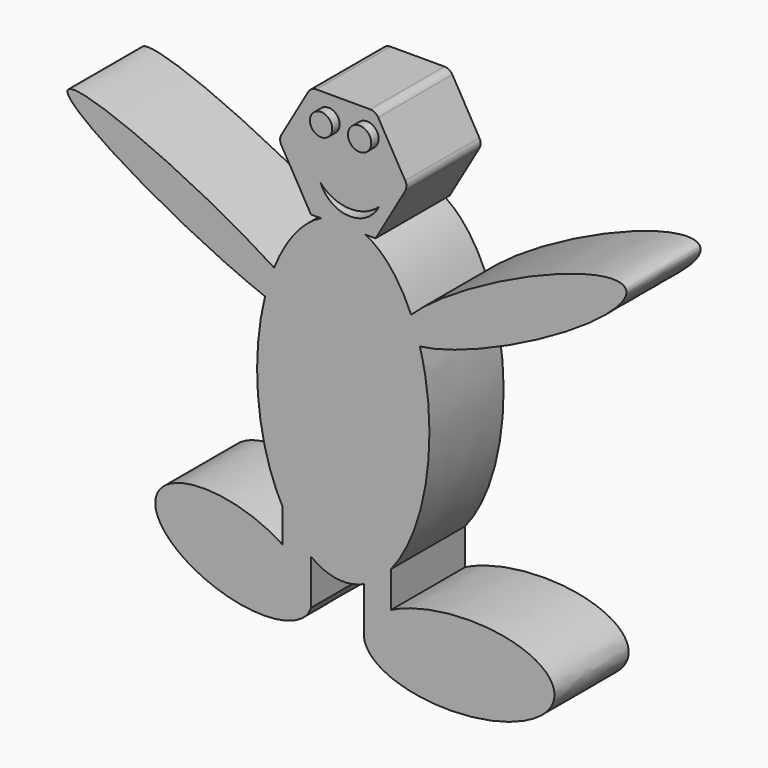
from build123d import *

# Parameters (mm, degrees)
F1_DEPTH = 50
F2_R     = 6.0155907658
F2_R_2   = 6.2756136539
F3_DEPTH = 5
F4_DEPTH = 10
F5_R     = 5
F7_DEPTH = 50


with BuildPart() as f1:
    # F0 (on Front) → F1 (new body)
    with BuildSketch(Plane.XZ):
        Polygon((17.4143397291, 30.1625211911), (-17.4143397291, 30.1625211911), (-34.8286794583, 0), (-17.4143397291, -30.1625211911), (17.4143397291, -30.1625211911), (34.8286794583, 0), align=None)
    extrude(amount=F1_DEPTH)

    # F2 (on face) → F3 (join)
    with BuildSketch(Plane.XZ.offset(50)):
        with Locations((-7.967392914, 17.6304206252)):
            Circle(F2_R)
        with Locations((12.811797671, 17.6304578781)):
            Circle(F2_R_2)
    extrude(amount=F3_DEPTH)

    # F2 (on face) → F4 (cut)
    with BuildSketch(Plane.XZ.offset(50)):
        with BuildLine():
            ThreePointArc((19.3255450577, -14.4387213513), (3.3384184901, -20.5933298221), (-12.2403670102, -13.468102552))
            ThreePointArc((-12.2403670102, -13.468102552), (3.2273641474, -24.2049759369), (19.3255450577, -14.4387213513))
        make_face()
    extrude(amount=-F4_DEPTH, mode=Mode.SUBTRACT)

    # F5
    f5_edges = [f1.edges().sort_by_distance(p)[0] for p in [
        (17.41434, -25, 30.162521),
        (-17.41434, -25, 30.162521),
        (34.828679, -25, 0),
        (-34.828679, -25, 0),
    ]]
    fillet(f5_edges, radius=F5_R)

    # F6 (on Front) → F7 (join)
    with BuildSketch(Plane.XZ):
        with BuildLine():
            add(Edge.make_bspline(
                [(41.2922416881, -73.6853662735), (169.4693590378, -59.4246752204), (152.5160927466, -10.667922077), (135.5628264553, 38.0888310665), (36.5988004625, -60.1872620557)],
                knots=[0.5054493336, 0.5054493336, 0.5054493336, 3.1146139618, 3.1146139618, 5.7237785899, 5.7237785899, 5.7237785899], degree=2, weights=[1, 0.2630807094, 1, 0.2630807094, 1]))
            add(Edge.make_bspline(
                [(41.2922416881, -73.6853662735), (39.2889405165, -66.529639937), (36.5988004625, -60.1872620557)],
                knots=[5.1892655065, 5.1892655065, 5.1892655065, 5.376524204, 5.376524204, 5.376524204], degree=2, weights=[1, 0.9956199737, 1]))
        make_face()
        with BuildLine():
            add(Edge.make_bspline(
                [(-37.2982655111, -61.8791791625), (-40.1784962307, -69.0282916237), (-42.20112137, -77.1171546989)],
                knots=[0.9314728887, 0.9314728887, 0.9314728887, 1.1384572321, 1.1384572321, 1.1384572321], degree=2, weights=[1, 0.9946494634, 1]))
            add(Edge.make_bspline(
                [(-37.2982655111, -61.8791791625), (-142.2676835981, 6.0363373075), (-148.6893936246, -13.9222058565), (-155.1111036512, -33.8807490205), (-42.20112137, -77.1171546989)],
                knots=[0.9261808498, 0.9261808498, 0.9261808498, 3.1635032717, 3.1635032717, 5.4008256936, 5.4008256936, 5.4008256936], degree=2, weights=[1, 0.4368871001, 1, 0.4368871001, 1]))
        make_face()
        with BuildLine():
            add(Edge.make_bspline(
                [(36.5988004625, -60.1872620557), (22.6424707083, -27.2832810879), (0, -27.2832810879)],
                knots=[5.376524204, 5.376524204, 5.376524204, 6.2831853072, 6.2831853072, 6.2831853072], degree=2, weights=[1, 0.8989934357, 1]))
            add(Edge.make_bspline(
                [(0, -27.2832810879), (-23.3602880424, -27.2832810879), (-37.2982655111, -61.8791791625)],
                knots=[0, 0, 0, 0.9314728887, 0.9314728887, 0.9314728887], degree=2, weights=[1, 0.8934910848, 1]))
            add(Edge.make_bspline(
                [(-14.1357605669, -82.8124405083), (-11.8424071187, -78.3491930143), (-37.2982655111, -61.8791791625)],
                knots=[0, 0, 0, 0.9261808498, 0.9261808498, 0.9261808498], degree=2, weights=[1, 0.8946762325, 1]))
            add(Edge.make_bspline(
                [(-42.20112137, -77.1171546989), (-16.3047277649, -87.0336116578), (-14.1357605669, -82.8124405083)],
                knots=[5.4008256936, 5.4008256936, 5.4008256936, 6.2831853072, 6.2831853072, 6.2831853072], degree=2, weights=[1, 0.9042485074, 1]))
            add(Edge.make_bspline(
                [(-42.20112137, -77.1171546989), (-55.8693379467, -131.7789554553), (-32.6593779027, -174.0816324883)],
                knots=[1.1384572321, 1.1384572321, 1.1384572321, 2.3624206627, 2.3624206627, 2.3624206627], degree=2, weights=[1, 0.8185111489, 1]))
            Line((-32.6593779027, -174.0816324883), (-32.6593779027, -169.5833057165))
            Line((-32.6593779027, -169.5833057165), (-17.4256470054, -169.5833057165))
            Line((-17.4256470054, -169.5833057165), (-17.4256470054, -192.5705769551))
            add(Edge.make_bspline(
                [(-17.4256470054, -192.5705769551), (-3.4362621433, -203.0115231159), (11.2084979191, -196.2957137528)],
                knots=[2.7572761224, 2.7572761224, 2.7572761224, 3.3851526537, 3.3851526537, 3.3851526537], degree=2, weights=[1, 0.9511247857, 1]))
            Line((11.2084979191, -196.2957137528), (11.2084979191, -181.6708147526))
            Line((11.2084979191, -181.6708147526), (25.7280766964, -181.6708147526))
            Line((25.7280766964, -181.6708147526), (25.7280766964, -184.4870319799))
            add(Edge.make_bspline(
                [(25.7280766964, -184.4870319799), (60.4040061865, -141.9519646735), (41.2922416881, -73.6853662735)],
                knots=[3.7282237262, 3.7282237262, 3.7282237262, 5.1892655065, 5.1892655065, 5.1892655065], degree=2, weights=[1, 0.7448269354, 1]))
            add(Edge.make_bspline(
                [(30.647560719, -71.4679593328), (32.2659775962, -74.6896076408), (41.2922416881, -73.6853662735)],
                knots=[0, 0, 0, 0.5054493336, 0.5054493336, 0.5054493336], degree=2, weights=[1, 0.9682347327, 1]))
            add(Edge.make_bspline(
                [(36.5988004625, -60.1872620557), (28.8474842086, -67.884696253), (30.647560719, -71.4679593328)],
                knots=[5.7237785899, 5.7237785899, 5.7237785899, 6.2831853072, 6.2831853072, 6.2831853072], degree=2, weights=[1, 0.9611373745, 1]))
        make_face()
        with BuildLine():
            add(Edge.make_bspline(
                [(41.2922416881, -73.6853662735), (39.2889405165, -66.529639937), (36.5988004625, -60.1872620557)],
                knots=[5.1892655065, 5.1892655065, 5.1892655065, 5.376524204, 5.376524204, 5.376524204], degree=2, weights=[1, 0.9956199737, 1]))
            add(Edge.make_bspline(
                [(36.5988004625, -60.1872620557), (28.8474842086, -67.884696253), (30.647560719, -71.4679593328)],
                knots=[5.7237785899, 5.7237785899, 5.7237785899, 6.2831853072, 6.2831853072, 6.2831853072], degree=2, weights=[1, 0.9611373745, 1]))
            add(Edge.make_bspline(
                [(30.647560719, -71.4679593328), (32.2659775962, -74.6896076408), (41.2922416881, -73.6853662735)],
                knots=[0, 0, 0, 0.5054493336, 0.5054493336, 0.5054493336], degree=2, weights=[1, 0.9682347327, 1]))
        make_face()
        with BuildLine():
            add(Edge.make_bspline(
                [(-14.1357605669, -82.8124405083), (-11.8424071187, -78.3491930143), (-37.2982655111, -61.8791791625)],
                knots=[0, 0, 0, 0.9261808498, 0.9261808498, 0.9261808498], degree=2, weights=[1, 0.8946762325, 1]))
            add(Edge.make_bspline(
                [(-37.2982655111, -61.8791791625), (-40.1784962307, -69.0282916237), (-42.20112137, -77.1171546989)],
                knots=[0.9314728887, 0.9314728887, 0.9314728887, 1.1384572321, 1.1384572321, 1.1384572321], degree=2, weights=[1, 0.9946494634, 1]))
            add(Edge.make_bspline(
                [(-42.20112137, -77.1171546989), (-16.3047277649, -87.0336116578), (-14.1357605669, -82.8124405083)],
                knots=[5.4008256936, 5.4008256936, 5.4008256936, 6.2831853072, 6.2831853072, 6.2831853072], degree=2, weights=[1, 0.9042485074, 1]))
        make_face()
        with BuildLine():
            Line((-32.6593779027, -169.5833057165), (-32.6593779027, -174.0816324883))
            add(Edge.make_bspline(
                [(-32.6593779027, -174.0816324883), (-26.0445481198, -186.1378793499), (-17.4256470054, -192.5705769551)],
                knots=[2.3624206627, 2.3624206627, 2.3624206627, 2.7572761224, 2.7572761224, 2.7572761224], degree=2, weights=[1, 0.9805743661, 1]))
            Line((-17.4256470054, -192.5705769551), (-17.4256470054, -169.5833057165))
            Line((-17.4256470054, -169.5833057165), (-32.6593779027, -169.5833057165))
        make_face()
        with BuildLine():
            add(Edge.make_bspline(
                [(-32.6593779027, -174.0816324883), (-26.0445481198, -186.1378793499), (-17.4256470054, -192.5705769551)],
                knots=[2.3624206627, 2.3624206627, 2.3624206627, 2.7572761224, 2.7572761224, 2.7572761224], degree=2, weights=[1, 0.9805743661, 1]))
            Line((-32.6593779027, -174.0816324883), (-32.6593779027, -191.9202000812))
            add(Edge.make_bspline(
                [(-17.4256470054, -209.6746091398), (-19.9783918544, -200.3396941884), (-32.6593779027, -191.9202000812)],
                knots=[0.3149352399, 0.3149352399, 0.3149352399, 1.0505459948, 1.0505459948, 1.0505459948], degree=2, weights=[1, 0.9331187091, 1]))
            Line((-17.4256470054, -209.6746091398), (-17.4256470054, -192.5705769551))
        make_face()
        with BuildLine():
            add(Edge.make_bspline(
                [(-17.4256470054, -209.6746091398), (-19.9783918544, -200.3396941884), (-32.6593779027, -191.9202000812)],
                knots=[0.3149352399, 0.3149352399, 0.3149352399, 1.0505459948, 1.0505459948, 1.0505459948], degree=2, weights=[1, 0.9331187091, 1]))
            Line((-32.6593779027, -191.9202000812), (-32.6593779027, -216.8934494257))
            Line((-32.6593779027, -216.8934494257), (-17.4256470054, -216.8934494257))
            Line((-17.4256470054, -216.8934494257), (-17.4256470054, -209.6746091398))
        make_face()
        with BuildLine():
            Line((-32.6593779027, -216.8934494257), (-32.6593779027, -191.9202000812))
            add(Edge.make_bspline(
                [(-32.6593779027, -191.9202000812), (-155.0656797466, -110.6489855928), (-98.566158617, -203.2708546887), (-42.0666374873, -295.8927237846), (-17.4256470054, -216.8934494257)],
                knots=[1.0505459948, 1.0505459948, 1.0505459948, 3.666865651, 3.666865651, 6.2831853072, 6.2831853072, 6.2831853072], degree=2, weights=[1, 0.2596275414, 1, 0.2596275414, 1]))
            Line((-17.4256470054, -216.8934494257), (-32.6593779027, -216.8934494257))
        make_face()
        with BuildLine():
            add(Edge.make_bspline(
                [(11.2084979191, -196.2957137528), (19.0225466962, -192.7123391043), (25.7280766964, -184.4870319799)],
                knots=[3.3851526537, 3.3851526537, 3.3851526537, 3.7282237262, 3.7282237262, 3.7282237262], degree=2, weights=[1, 0.9853238194, 1]))
            Line((25.7280766964, -184.4870319799), (25.7280766964, -181.6708147526))
            Line((25.7280766964, -181.6708147526), (11.2084979191, -181.6708147526))
            Line((11.2084979191, -181.6708147526), (11.2084979191, -196.2957137528))
        make_face()
        with BuildLine():
            Line((25.7280766964, -203.876795604), (25.7280766964, -184.4870319799))
            add(Edge.make_bspline(
                [(11.2084979191, -196.2957137528), (19.0225466962, -192.7123391043), (25.7280766964, -184.4870319799)],
                knots=[3.3851526537, 3.3851526537, 3.3851526537, 3.7282237262, 3.7282237262, 3.7282237262], degree=2, weights=[1, 0.9853238194, 1]))
            Line((11.2084979191, -196.2957137528), (11.2084979191, -219.9759412186))
            add(Edge.make_bspline(
                [(25.7280766964, -203.876795604), (11.7578588698, -210.9900355862), (11.2084979191, -219.9759412186)],
                knots=[5.4843672103, 5.4843672103, 5.4843672103, 6.2283501589, 6.2283501589, 6.2283501589], degree=2, weights=[1, 0.9316053495, 1]))
        make_face()
        with BuildLine():
            Line((25.7280766964, -221.2353944778), (25.7280766964, -203.876795604))
            add(Edge.make_bspline(
                [(25.7280766964, -203.876795604), (11.7578588698, -210.9900355862), (11.2084979191, -219.9759412186)],
                knots=[5.4843672103, 5.4843672103, 5.4843672103, 6.2283501589, 6.2283501589, 6.2283501589], degree=2, weights=[1, 0.9316053495, 1]))
            Line((11.2084979191, -219.9759412186), (11.2084979191, -221.2353944778))
            Line((11.2084979191, -221.2353944778), (25.7280766964, -221.2353944778))
        make_face()
        with BuildLine():
            add(Edge.make_bspline(
                [(11.2084979191, -221.2353944778), (13.0350369218, -250.9322399042), (76.9798142406, -239.4129351389), (140.9245915595, -227.8936303736), (106.5507257658, -204.0600093155), (72.1768599722, -180.2263882575), (25.7280766964, -203.876795604)],
                knots=[0, 0, 0, 1.8281224034, 1.8281224034, 3.6562448069, 3.6562448069, 5.4843672103, 5.4843672103, 5.4843672103], degree=2, weights=[1, 0.610534363, 1, 0.610534363, 1, 0.610534363, 1]))
            Line((25.7280766964, -203.876795604), (25.7280766964, -221.2353944778))
            Line((25.7280766964, -221.2353944778), (11.2084979191, -221.2353944778))
        make_face()
    extrude(amount=F7_DEPTH)


solid = f1.part
